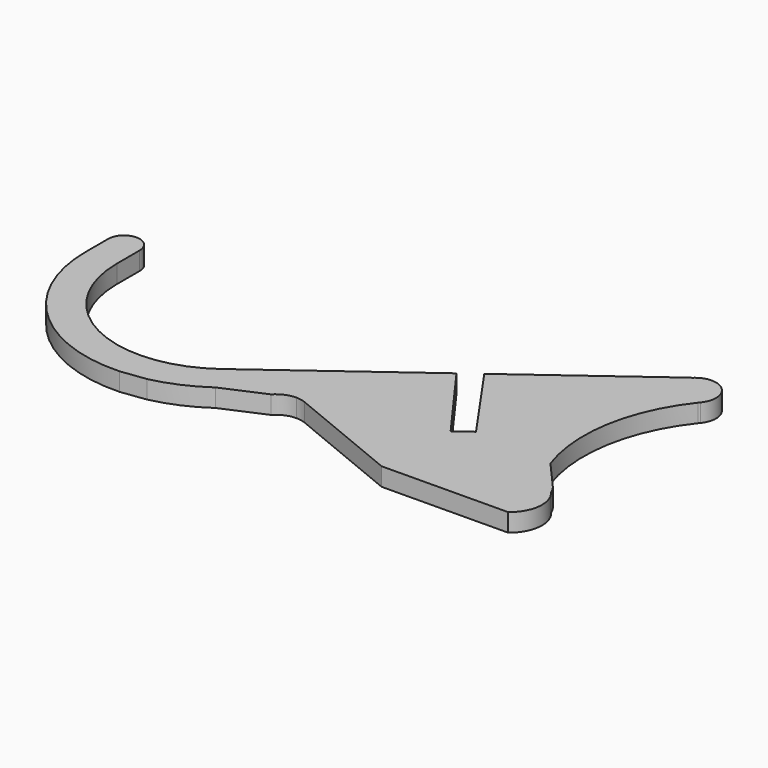
from build123d import *

# Parameters (mm, degrees)
F1_DEPTH = 6.35
F3_DEPTH = 6.351


with BuildPart() as f1:
    # F0 (on Top) → F1 (new body)
    with BuildSketch(Plane.XY):
        with BuildLine():
            Line((64.0479785321, 45.3746123328), (63.8854764337, 45.3746123328))
            Line((63.8854764337, 45.3746123328), (2.2767815665, 0))
            Line((2.2767815665, 0), (-39.7214530308, -30.9315692797))
            ThreePointArc((-39.7214530308, -30.9315692797), (-39.8444384128, -31.0225247493), (-39.9677839364, -31.1129912262))
            ThreePointArc((-39.9677839364, -31.1129912262), (-80.1407322996, -34.3509043357), (-101.2207046151, 0))
            Line((-101.2207046151, 0), (-101.2207046151, 9.9341273308))
            ThreePointArc((-101.2207046151, 9.9341273308), (-106.7247502506, 15.4381729662), (-112.228795886, 9.9341273308))
            Line((-112.228795886, 9.9341273308), (-112.228795886, 0))
            ThreePointArc((-112.228795886, 0), (-97.0433078129, -35.6915315199), (-60.7969101261, -49.5003375864))
            Line((-60.7969101261, -49.5003375864), (-52.0564235031, -48.3813164917))
            ThreePointArc((-52.0564235031, -48.3813164917), (-42.7531679645, -45.3464600069), (-34.228034924, -40.5419804156))
            Line((-34.228034924, -40.5419804156), (-34.2284778363, -40.5419804156))
            Line((-34.2284778363, -40.5419804156), (-34.2273214057, -40.5414794451))
            Line((-34.2273214057, -40.5414794451), (-19.8154687348, -34.2982047457))
            ThreePointArc((-19.8154687348, -34.2982047457), (-16.7847778238, -32.1655358704), (-13.1560671025, -31.4133241773))
            ThreePointArc((-13.1560671025, -31.4133241773), (-11.5145721435, -31.5621218969), (-9.9265901442, -32.0036642296))
            Line((-9.9265901442, -32.0036642296), (30.5177745747, -48.6430156736))
            Line((30.5177745747, -48.6430156736), (74.522745552, -48.229868259))
            ThreePointArc((74.522745552, -48.229868259), (79.0697257066, -40.3110135201), (76.337517689, -31.5979010883))
            ThreePointArc((76.337517689, -31.5979010883), (75.6238074008, -30.083288758), (74.6402267249, -28.7282972671))
            Line((74.6402267249, -28.7282972671), (65.5481898023, -18.39660376))
            ThreePointArc((65.5481898023, -18.39660376), (63.2520758801, 9.4447724115), (74.6402267249, 34.9540724138))
            Line((74.6402267249, 34.9540724138), (74.6402267249, 35.0096798031))
            ThreePointArc((74.6402267249, 35.0096798031), (74.8701460848, 35.255569914), (75.088660103, 35.5116489692))
            ThreePointArc((75.088660103, 35.5116489692), (74.2807317817, 45.7182435688), (64.0479785321, 45.3746123328))
        make_face()
    extrude(amount=F1_DEPTH)

    # F2 (on face) → F3 (cut, through all)
    with BuildSketch(Plane.XY.offset(6.35)):
        Polygon((12.0820117015, 7.2215215266), (32.3011358824, -20.6074602199), (37.9280887206, -16.5192021861), (18.2175485278, 11.7403253342), align=None)
    extrude(amount=-F3_DEPTH, mode=Mode.SUBTRACT)


solid = f1.part
